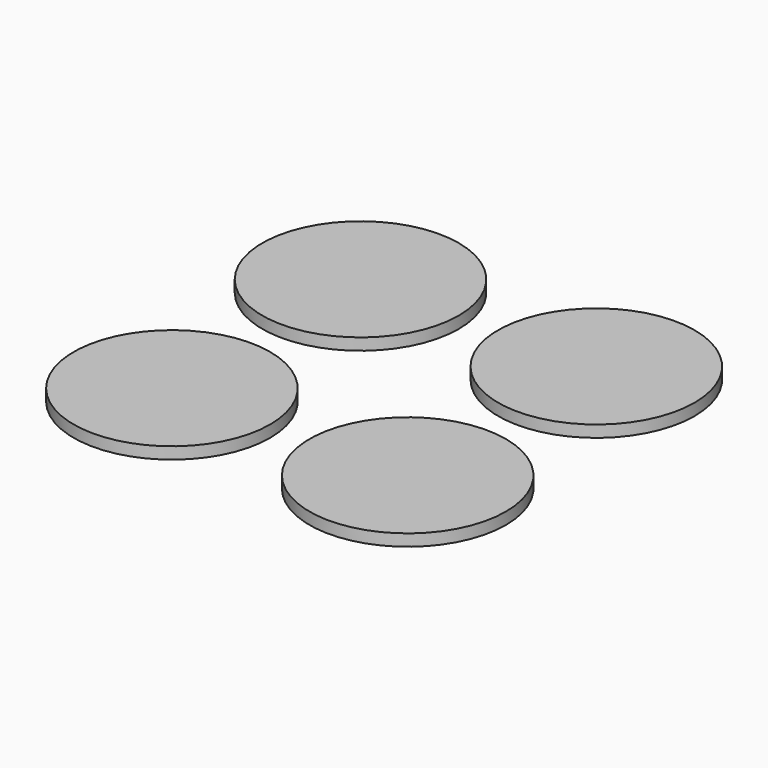
from build123d import *

# Parameters (mm, degrees)
F0_R         = 50
F1_DEPTH     = 6
F2_TEXT_SIZE = 11.8273939693
F3_DEPTH     = 2
F4_TEXT_SIZE = 7.4849747545
F5_DEPTH     = 2


# Not quite as in the source:
# - Text() gives the source's letters only with a copy of the font that has no kerning and outlines rounded to 1/6400 em; it was checked with that copy


with BuildPart() as f1:
    # F0 (on Top) → F1 (new body)
    with BuildSketch(Plane.XY):
        Circle(F0_R)
    extrude(amount=F1_DEPTH)

    # F2 (on face) → F3 (cut)
    with BuildSketch(Plane(origin=(0, 0, 0), x_dir=(1, 0, 0), z_dir=(0, 0, -1))):
        with Locations((-30, -4.2657236579)):
            Text('MIROCOLS', F2_TEXT_SIZE, font='Open Sans', text_align=(TextAlign.LEFT, TextAlign.BOTTOM))
    extrude(amount=-F3_DEPTH, mode=Mode.SUBTRACT)

    # F4 (on face) → F5 (cut)
    with BuildSketch(Plane(origin=(0, 0, 0), x_dir=(1, 0, 0), z_dir=(0, 0, -1))):
        with Locations((-15.2933238089, -15.4210680462)):
            Text('Coasters', F4_TEXT_SIZE, font='Open Sans', text_align=(TextAlign.LEFT, TextAlign.BOTTOM))
    extrude(amount=-F5_DEPTH, mode=Mode.SUBTRACT)


with BuildPart() as f6_1:
    # F6: copy of F1
    add(f1.part.moved(Location((120, 0, 0))))


with BuildPart() as f7_1:
    # F7: copy of F1
    add(f1.part.moved(Location((0, 120, 0))))


with BuildPart() as f8_1:
    # F8: copy of F6_1
    add(f6_1.part.moved(Location((0, 120, 0))))


solid = Compound([f1.part, f6_1.part, f7_1.part, f8_1.part])
